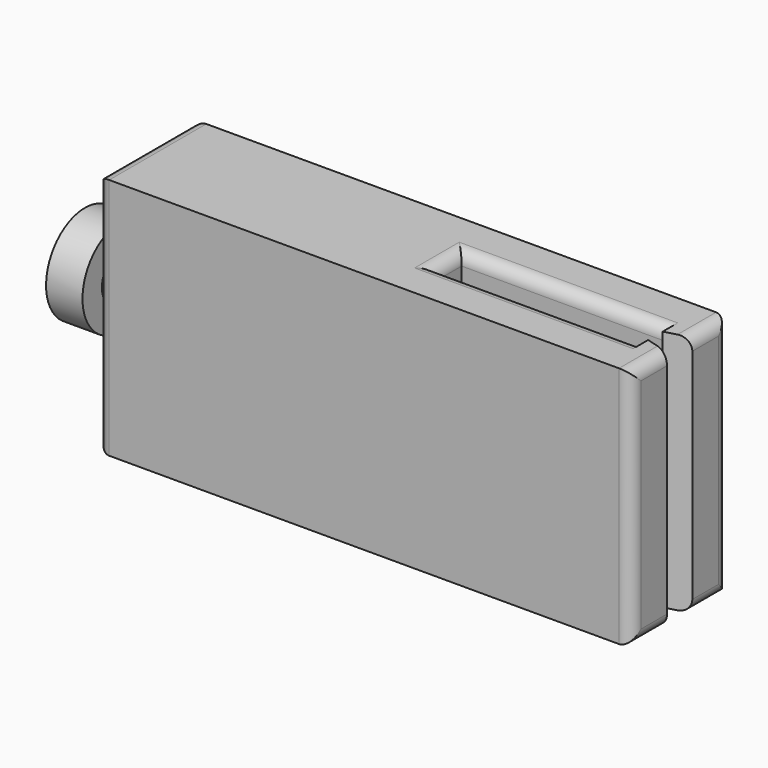
from build123d import *

# Parameters (mm, degrees)
F1_DEPTH = 10
F2_R     = 2
F3_DEPTH = 2
F4_R     = 4
F4_R_2   = 2
F5_DEPTH = 3
F6_R     = 1
F7_ANGLE = 90


# Not quite as in the source:
# - a feature names something its author has since deleted; it is built from what else it names


with BuildPart() as f1:
    # F0 (on Front) → F1 (new body, symmetric)
    with BuildSketch(Plane.XZ):
        Polygon((0, 5), (0, 0), (25, 0), (25, 1.3), (25, 5), align=None)
        Polygon((25, 0), (0, 0), (0, -5), (25, -5), (25, -1.3), align=None)
        Polygon((25, 5), (25, 1.3), (42, 1.3), (44, 1.3), (44, 5), align=None)
        Polygon((42, -1.3), (25, -1.3), (25, -5), (44, -5), (44, -1.3), align=None)
        Polygon((44, 1.3), (42, 1.3), (42, 0.75), align=None)
        Polygon((42, -0.75), (42, -1.3), (44, -1.3), align=None)
    extrude(amount=F1_DEPTH, both=True)

    # F2 (on face) → F3 (join)
    with BuildSketch(Plane(origin=(0, 0, 0), x_dir=(0, -1, 0), z_dir=(-1, 0, 0))):
        Circle(F2_R)
    extrude(amount=F3_DEPTH)

    # F4 (on face) → F5 (join)
    with BuildSketch(Plane(origin=(-2, 0, 0), x_dir=(0, -1, 0), z_dir=(-1, 0, 0))):
        Circle(F4_R)
        Circle(F4_R_2, mode=Mode.SUBTRACT)
        Circle(F4_R_2)
    extrude(amount=F5_DEPTH)

    # F6
    f6_edges = [f1.edges().sort_by_distance(p)[0] for p in [
        (44, -10, 3.15),
        (44, 10, 3.15),
        (44, 10, -3.15),
        (44, -10, -3.15),
        (0, -10, 0),
        (0, 10, 0),
        (0, 0, 5),
        (0, 0, -5),
        (44, 0, -5),
        (44, 0, 5),
        (33.5, -10, 1.3),
        (33.5, -10, -1.3),
        (25, -10, 0),
        (25, 10, 0),
        (33.5, 10, 1.3),
        (33.5, 10, -1.3),
    ]]
    fillet(f6_edges, radius=F6_R)


with BuildPart() as f1_1:
    # F7: moved
    add(f1.part.rotate(Axis((12.5, 0, 0), (1, 0, 0)), F7_ANGLE))


solid = f1_1.part
